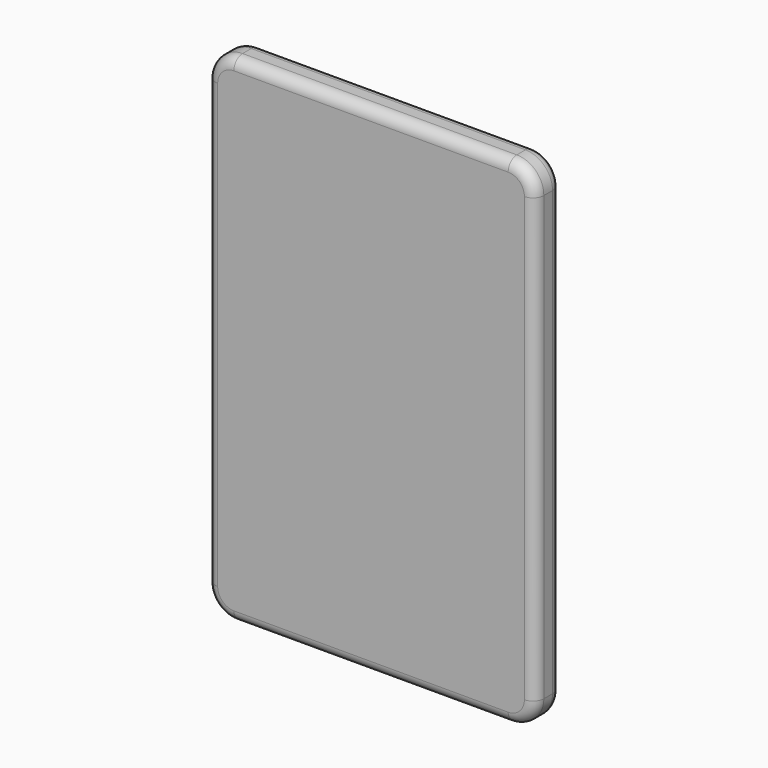
from build123d import *

# Parameters (mm, degrees)
F0_W     = 154.28596735
F0_H     = 233.5498631001
F2_DEPTH = 15.24
F3_DEPTH = 15.24
F4_R     = 12.7
F6_R     = 12.7
F7_R     = 12.7
F8_R     = 12.7
F9_R     = 5.08


# Not quite as in the source:
# - the program builds the solid bodies; features that only make, move or delete a surface that nothing else refers to are left out


with BuildPart() as f2:
    # F0 (on Front) → F2 (new body)
    with BuildSketch(Plane.XZ):
        Rectangle(F0_W, F0_H)
    extrude(amount=-F2_DEPTH)

    # F3 (add): a face of the model
    f3_faces = [f2.faces().sort_by_distance(p)[0] for p in [
        (0, 15.24, 0),
    ]]
    extrude(f3_faces, amount=-F3_DEPTH)

    # F4
    f4_edges = [f2.edges().sort_by_distance(p)[0] for p in [
        (77.142984, 7.62, 116.774932),
    ]]
    fillet(f4_edges, radius=F4_R)

    # F6
    f6_edges = [f2.edges().sort_by_distance(p)[0] for p in [
        (-77.142984, 7.62, 116.774932),
    ]]
    fillet(f6_edges, radius=F6_R)

    # F7
    f7_edges = [f2.edges().sort_by_distance(p)[0] for p in [
        (77.142984, 7.62, -116.774932),
    ]]
    fillet(f7_edges, radius=F7_R)

    # F8
    f8_edges = [f2.edges().sort_by_distance(p)[0] for p in [
        (-77.142984, 7.62, -116.774932),
    ]]
    fillet(f8_edges, radius=F8_R)

    # F9
    f9_edges = [f2.edges().sort_by_distance(p)[0] for p in [
        (-77.142984, 15.24, 0),
        (-77.142984, 0, 0),
        (77.142984, 0, 0),
        (77.142984, 15.24, 0),
        (0, 0, 116.774932),
        (0, 15.24, 116.774932),
        (0, 15.24, -116.774932),
        (0, 0, -116.774932),
    ]]
    fillet(f9_edges, radius=F9_R)


solid = f2.part
